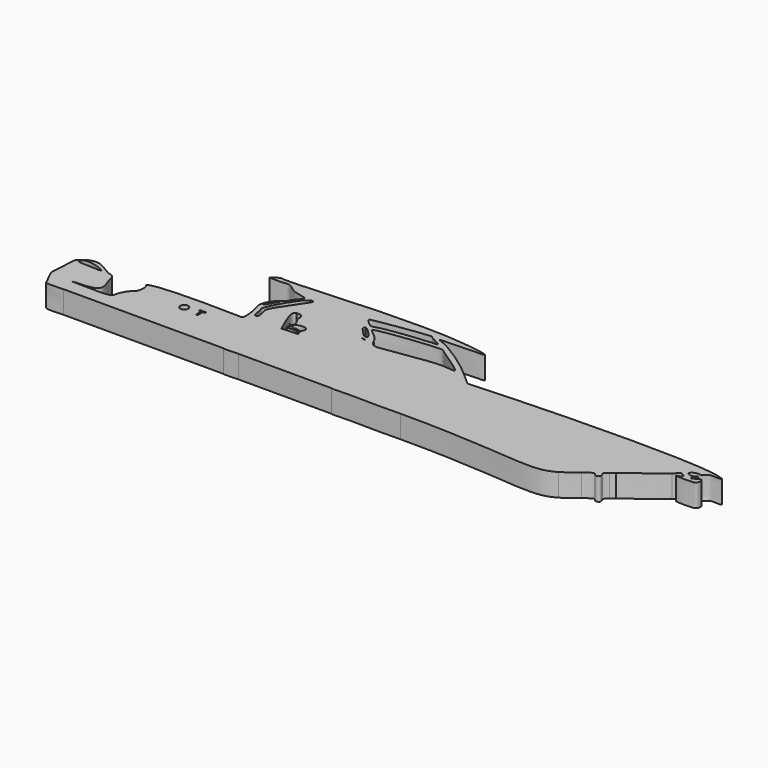
from build123d import *

# Parameters (mm, degrees)
F0_R     = 1.735828002
F1_DEPTH = 9.906


# Not quite as in the source:
# - a feature names something its author has since deleted; it is built from what else it names


with BuildPart() as f1:
    # F0 (on Top) → F1 (new body)
    with BuildSketch(Plane.XY):
        with BuildLine():
            add(Edge.make_bspline(
                [(181.7070857524, 12.9581492726), (181.3160846649, 13.0694763777), (171.7126869599, 17.0451590909), (106.450533251, 15.778155012), (69.6900859475, 13.5057969019)],
                knots=[0.0181687305, 0.0181687305, 0.0181687305, 0.0181687305, 0.0992372423, 0.5806503873, 0.5806503873, 0.5806503873, 0.5806503873], degree=3))
            add(Edge.make_bspline(
                [(69.6900859475, 13.5057969019), (46.0973907721, 12.0474073514), (24.7516413203, 9.403863054), (23.4549589902, 8.8764271796), (19.9190564454, 8.5168434307)],
                knots=[0.5806503873, 0.5806503873, 0.5806503873, 0.5806503873, 0.8896192497, 1, 1, 1, 1], degree=3))
            add(Edge.make_bspline(
                [(19.9190564454, 8.5168434307), (17.4676650102, 8.1993707105), (12.0162404463, 7.4933722476), (-0.135088308, 4.7670167299), (-6.1064609958, 3.2006267697), (-14.1477540249, 3.5424096416), (-21.6224677861, 3.7269103341)],
                knots=[0, 0, 0, 0, 0.0359936003, 0.0800441177, 0.1106409376, 0.1609466089, 0.1609466089, 0.1609466089, 0.1609466089], degree=3))
            add(Edge.make_bspline(
                [(-21.6224677861, 3.7269103341), (-32.9219585505, 4.005819191), (-55.8180186536, 4.2959920551), (-62.3599502161, 2.2052144497), (-62.1269792318, 1.8509117654)],
                knots=[0.1609466089, 0.1609466089, 0.1609466089, 0.1609466089, 0.236993463, 0.2636435799, 0.2636435799, 0.2636435799, 0.2636435799], degree=3))
            add(Edge.make_bspline(
                [(-62.1269792318, 1.8509117654), (-62.1143161054, 1.8367462376), (-62.101652979, 1.8225807098), (-62.0890020197, 1.8083766563)],
                knots=[0, 0, 0, 0, 0.0040737181, 0.0040737181, 0.0040737181, 0.0040737181], degree=3))
            add(Edge.make_bspline(
                [(-62.0890020197, 1.8083766563), (-61.861903726, 1.6076355151), (-60.1495223277, 1.3262390965), (-58.7832820227, 0.8461268043), (-52.5991049945, 0.8259101603), (-44.5873551936, 0.8045360783), (-38.4716986515, 0.9143963036), (-28.4774091761, 1.0996765249), (-16.1932718144, 0.7142595445), (-10.6895341404, 0.9946984772), (-5.449048277, 0.7670292415), (-2.858249547, 1.3382218789), (0.1983725594, 2.3648289955), (1.4864198165, 2.7889108751)],
                knots=[0.2647332889, 0.2647332889, 0.2647332889, 0.2647332889, 0.2804985871, 0.296751932, 0.3273978904, 0.3637260288, 0.3948079699, 0.4350461602, 0.4794644674, 0.5096583468, 0.5375063976, 0.558553087, 0.585278667, 0.585278667, 0.585278667, 0.585278667], degree=3))
            add(Edge.make_bspline(
                [(1.4864198165, 2.7889108751), (2.5730539489, 3.1466786843), (4.4584634209, 3.748123171), (10.8733523881, 4.5985160145), (15.272056911, 5.6548268597), (21.1046291923, 6.5191676625), (28.0641113783, 7.5548859125), (52.7585985721, 10.7246110457), (65.7444362113, 10.6342542254), (72.0763572093, 11.8721236252), (132.1513691778, 12.467602904), (181.7070857524, 12.9581492726)],
                knots=[0.585278667, 0.585278667, 0.585278667, 0.585278667, 0.6078251436, 0.6393387701, 0.6669634416, 0.6961942967, 0.7301717216, 0.793934581, 0.8383697732, 0.8667529058, 0.9998969364, 0.9998969364, 0.9998969364, 0.9998969364], degree=3))
        make_face()
        with BuildLine():
            add(Edge.make_bspline(
                [(69.6900859475, 13.5057969019), (46.0973907721, 12.0474073514), (24.7516413203, 9.403863054), (23.4549589902, 8.8764271796), (19.9190564454, 8.5168434307)],
                knots=[0.5806503873, 0.5806503873, 0.5806503873, 0.5806503873, 0.8896192497, 1, 1, 1, 1], degree=3))
            add(Edge.make_bspline(
                [(-32.5296521187, 32.6141417027), (-31.3157910097, 33.5724732534), (-29.3571477605, 35.1188029908), (-27.6202321809, 34.0767531544), (0.8249259172, 36.2700535088), (31.2175375693, 37.1804566476), (49.4536321074, 36.4065733844), (69.3127565879, 32.985000615), (38.7618020948, 33.6435412252), (44.2668843403, 32.1137581005), (51.7651660713, 27.9376072981), (61.6112530423, 20.8457781991), (67.040172836, 15.8285102723), (69.6900859475, 13.5057969019)],
                knots=[0, 0, 0, 0, 0.0527292582, 0.0850128218, 0.2240344771, 0.3801343496, 0.5042178826, 0.5822497204, 0.6998266016, 0.7329381334, 0.8150611757, 0.9107169826, 1, 1, 1, 1], degree=3))
            add(Edge.make_bspline(
                [(-32.5296521187, 32.6141417027), (-30.3104056847, 32.52847609), (-26.5690998673, 32.391920198), (-23.2049727281, 33.2819990285), (-19.7617512793, 28.9993191577), (-10.3988767952, 28.7616312209), (-16.2720736116, 25.3132861108), (-16.9129986316, 22.6762704551)],
                knots=[0, 0, 0, 0, 0.2160762386, 0.3662971417, 0.569378152, 0.7796526031, 1, 1, 1, 1], degree=3))
            add(Edge.make_bspline(
                [(-16.9129986316, 22.6762704551), (-17.8467477386, 22.1680560361), (-19.9763271995, 21.0089834539), (-23.3696805255, 15.5020605961), (-21.7713441225, 12.3045577284), (-20.779820899, 4.7533250441), (-21.4380773918, 3.9515133273), (-21.6224677861, 3.7269103341)],
                knots=[0, 0, 0, 0, 0.1877547788, 0.4282078748, 0.6241699663, 0.8947227276, 1, 1, 1, 1], degree=3))
            add(Edge.make_bspline(
                [(19.9190564454, 8.5168434307), (17.4676650102, 8.1993707105), (12.0162404463, 7.4933722476), (-0.135088308, 4.7670167299), (-6.1064609958, 3.2006267697), (-14.1477540249, 3.5424096416), (-21.6224677861, 3.7269103341)],
                knots=[0, 0, 0, 0, 0.0359936003, 0.0800441177, 0.1106409376, 0.1609466089, 0.1609466089, 0.1609466089, 0.1609466089], degree=3))
        make_face()
        with BuildLine():
            add(Edge.make_bspline(
                [(-8.7680807337, 17.8092923015), (-8.3866222979, 17.8483506489), (-7.546092961, 17.9344142503), (-5.9981024532, 17.2405624552), (-5.6060574812, 15.7239200529), (-6.0102153242, 14.5268353778), (-5.4550952735, 13.7705655392), (-4.6619934349, 12.9765246302), (-4.4702294547, 12.3041590957), (-4.0660592451, 10.8605465604), (-4.3298750077, 9.9418295588), (-5.4584476986, 9.754342472), (-5.6748329949, 10.4291802539), (-5.6347727128, 9.3913742433), (-4.3029010056, 9.7861895365), (-4.3140752557, 8.9878988444), (-4.4250907254, 8.1865468653), (-5.1640550787, 7.5215406766), (-4.3832359422, 7.2748261031), (-3.3321553041, 7.4747711988), (-2.8663373676, 7.4992743174), (-2.115136075, 7.4933709617), (-0.8968103525, 7.1797893281), (-1.5445606345, 7.8573288432), (-1.310513294, 9.0220769068), (-2.6227539696, 8.3145975273), (-3.1977834194, 8.2778539141), (-3.4696750478, 8.9956573412), (-4.0448585774, 9.7693814037), (-3.9314235683, 10.394370376), (-3.4871454114, 10.8062850186), (-2.8829533176, 11.0326311001), (-2.4154737172, 11.2246835665), (-2.3047583969, 11.3243672691), (-1.5621432493, 11.3791968524), (-0.7704961294, 11.3668207714), (0.0011303932, 11.2391718235), (0.2761138653, 11.255904495), (0.9514057607, 11.01202914), (1.2073443869, 10.382397098), (1.4002015739, 9.6657434855), (1.0307265988, 8.9530975397), (0.7733677818, 8.2984308224), (-0.4727618848, 7.7586873364), (-0.8225833851, 9.2751421466), (-0.4934208188, 7.4734539438), (0.0075581501, 7.445925416), (0.3338729219, 7.68534912), (0.9549221847, 7.2664605316), (1.3294265015, 6.722294157), (1.2187918234, 6.2131527361), (1.1623987395, 5.9606525059)],
                knots=[0, 0, 0, 0, 0.0260454786, 0.0555593992, 0.0840154219, 0.1096289478, 0.1317188239, 0.1562843989, 0.1764181206, 0.2050873592, 0.2270500346, 0.249871093, 0.2633196669, 0.2802385774, 0.3041836822, 0.3215813241, 0.3439096138, 0.3640338166, 0.3813082826, 0.4062842171, 0.4223932343, 0.4439778086, 0.4659830297, 0.4836895774, 0.5050499879, 0.5297363334, 0.5468542516, 0.5664129357, 0.5896734041, 0.6073348608, 0.6252199, 0.644737738, 0.6610014027, 0.6698170215, 0.6893495641, 0.7117052382, 0.7320089542, 0.7446274286, 0.7635758386, 0.7829107313, 0.8029010202, 0.8234292288, 0.84378532, 0.8679512846, 0.8872861973, 0.9123156375, 0.9274517817, 0.9412478508, 0.9605987473, 0.9795496341, 1, 1, 1, 1], degree=3))
            add(Edge.make_bspline(
                [(1.1623987395, 5.9606525059), (-1.3945692664, 5.7893390901), (-5.1543167158, 5.7216326818), (-5.4948480663, 5.4527658301), (-5.6129922159, 5.3594848141)],
                knots=[0.9337593868, 0.9337593868, 0.9337593868, 0.9337593868, 0.9769868279, 1, 1, 1, 1], degree=3))
            add(Edge.make_bspline(
                [(-8.7680807337, 17.8092923015), (-9.1752028405, 17.6145650541), (-10.8178823014, 16.8288684671), (-7.8473254678, 10.2830134292), (-5.6129922159, 5.3594848141)],
                knots=[0, 0, 0, 0, 0.2478402613, 1, 1, 1, 1], degree=3))
        make_face(mode=Mode.SUBTRACT)
        with BuildLine():
            add(Edge.make_bspline(
                [(-18.4361021966, 21.1632531136), (-18.5670530022, 21.2586161996), (-21.070472051, 18.5655291506), (-22.3743986232, 16.3744597495), (-21.4413586586, 15.2038485553), (-20.4225931001, 17.854661305), (-18.2993558507, 21.0636695068), (-18.4361021966, 21.1632531136)],
                knots=[0, 0, 0, 0, 0.2351165364, 0.4465883524, 0.5497009663, 0.7544778204, 1, 1, 1, 1], degree=3))
        make_face(mode=Mode.SUBTRACT)
        with BuildLine():
            add(Edge.make_bspline(
                [(-9.7060799599, 27.9816947877), (-9.8874931048, 28.2447168603), (-12.368524278, 29.356752937), (-21.4951287489, 13.0755897254), (-19.6376283471, 12.2112957368), (-19.6141174394, 7.2221985209), (-17.0553430775, 7.6758488961), (-18.6586504228, 11.9438536073), (-18.5103546144, 13.6291611502), (-17.1677183959, 16.6289965217), (-10.000495834, 26.8513547323), (-9.5698072007, 27.7841195592), (-9.7060799599, 27.9816947877)],
                knots=[0, 0, 0, 0, 0.0653917324, 0.2773427404, 0.3459565689, 0.4503618884, 0.5044288692, 0.6067460895, 0.6730479064, 0.7686451707, 0.9508794591, 1, 1, 1, 1], degree=3))
        make_face(mode=Mode.SUBTRACT)
        with BuildLine():
            add(Edge.make_bspline(
                [(22.0193362931, 17.0219166161), (21.0430994165, 17.2670474431), (19.9439292923, 17.5707458095), (19.3718951195, 17.5534747541)],
                knots=[0.6042790893, 0.6042790893, 0.6042790893, 0.6042790893, 0.632909986, 0.632909986, 0.632909986, 0.632909986], degree=3))
            add(Edge.make_bspline(
                [(22.0193362931, 17.0219166161), (21.930461642, 16.7429022187), (20.6518410174, 17.150070539), (19.3718951195, 17.5534747541)],
                knots=[0.9338982102, 0.9338982102, 0.9338982102, 0.9338982102, 1, 1, 1, 1], degree=3))
        make_face(mode=Mode.SUBTRACT)
        with BuildLine():
            add(Edge.make_bspline(
                [(19.099231914, 19.6574293824), (19.2141128722, 19.559261403), (19.3324185741, 19.4665098594), (19.4542166063, 19.3811532624)],
                knots=[0.4773801215, 0.4773801215, 0.4773801215, 0.4773801215, 0.5030785781, 0.5030785781, 0.5030785781, 0.5030785781], degree=3))
            add(Edge.make_bspline(
                [(16.2104386836, 24.2807362229), (15.7704996157, 24.2210769069), (16.1269574289, 22.4635564191), (17.0786160293, 22.2094376386), (18.2129434355, 20.4147798645), (19.099231914, 19.6574293824)],
                knots=[0, 0, 0, 0, 0.1478459221, 0.2791205811, 0.4773801215, 0.4773801215, 0.4773801215, 0.4773801215], degree=3))
            add(Edge.make_bspline(
                [(21.0577676507, 18.8489194134), (21.20328979, 18.8904985397), (21.8588734633, 19.6430869693), (17.1846356138, 24.4128452505), (16.2104386836, 24.2807362229)],
                knots=[0.6228285443, 0.6228285443, 0.6228285443, 0.6228285443, 0.672611382, 1, 1, 1, 1], degree=3))
            add(Edge.make_bspline(
                [(19.649869615, 19.2525507144), (20.1684843746, 18.9343377038), (20.7473442621, 18.7602240898), (21.0577676507, 18.8489194134)],
                knots=[0.5166333136, 0.5166333136, 0.5166333136, 0.5166333136, 0.6228285443, 0.6228285443, 0.6228285443, 0.6228285443], degree=3))
            add(Edge.make_bspline(
                [(19.4542166063, 19.3811532624), (19.5194574132, 19.3351449211), (19.5846240735, 19.2921451484), (19.649869615, 19.2525507144)],
                knots=[0.4893319279, 0.4893319279, 0.4893319279, 0.4893319279, 0.4932270857, 0.4932270857, 0.4932270857, 0.4932270857], degree=3))
        make_face(mode=Mode.SUBTRACT)
        with BuildLine():
            add(Edge.make_bspline(
                [(26.768874377, 15.5890742317), (28.477421113, 14.8122982972), (35.2147378262, 16.493420054), (41.3114742367, 16.8146107371), (54.2220403717, 19.4096476067), (64.7203055195, 16.7217366675), (47.1864971217, 27.407686439), (47.969181218, 28.4052858834), (17.3145197031, 25.37667601), (19.9733974533, 23.3131590908), (22.3191658115, 21.5089275881), (24.8989437371, 18.7282663545), (25.6097683501, 16.1160517198), (26.768874377, 15.5890742317)],
                knots=[0, 0, 0, 0, 0.0984646732, 0.1912591061, 0.323936191, 0.3995561971, 0.5344920224, 0.5848516391, 0.76862153, 0.8014841712, 0.8639750777, 0.9331999566, 1, 1, 1, 1], degree=3))
        make_face(mode=Mode.SUBTRACT)
        with BuildLine():
            add(Edge.make_bspline(
                [(13.7598691508, 29.2401816696), (14.0794886419, 28.511657453), (16.931970818, 25.6172264089), (19.0667686569, 26.8110867482), (27.6858636418, 28.3987828014), (40.9320979411, 29.6761274961), (44.8001711563, 29.781861299), (38.0692510724, 32.9302009921), (38.7545990359, 33.7239035632), (14.6777023437, 30.2669926278), (13.5969193313, 29.6116011009), (13.7598691508, 29.2401816696)],
                knots=[0, 0, 0, 0, 0.1009240569, 0.1708567082, 0.3169576193, 0.502818054, 0.5609304523, 0.6778465933, 0.710253389, 0.9485464519, 1, 1, 1, 1], degree=3))
        make_face(mode=Mode.SUBTRACT)
        with BuildLine():
            add(Edge.make_bspline(
                [(181.7070857524, 12.9581492726), (181.7454456589, 12.958528993), (181.7838055875, 12.9589087131), (181.8221655209, 12.9592884332)],
                knots=[0.9998969364, 0.9998969364, 0.9998969364, 0.9998969364, 1, 1, 1, 1], degree=3))
            add(Edge.make_bspline(
                [(181.8221655209, 12.9592884332), (181.8324633094, 12.9314378649), (181.7947152553, 12.9331991147), (181.7070857524, 12.9581492726)],
                knots=[0, 0, 0, 0, 0.0181687305, 0.0181687305, 0.0181687305, 0.0181687305], degree=3))
        make_face()
        with BuildLine():
            add(Edge.make_bspline(
                [(181.8221655209, 12.9592884332), (181.8324633094, 12.9314378649), (181.7947152553, 12.9331991147), (181.7070857524, 12.9581492726)],
                knots=[0, 0, 0, 0, 0.0181687305, 0.0181687305, 0.0181687305, 0.0181687305], degree=3))
            add(Edge.make_bspline(
                [(1.4864198165, 2.7889108751), (2.5730539489, 3.1466786843), (4.4584634209, 3.748123171), (10.8733523881, 4.5985160145), (15.272056911, 5.6548268597), (21.1046291923, 6.5191676625), (28.0641113783, 7.5548859125), (52.7585985721, 10.7246110457), (65.7444362113, 10.6342542254), (72.0763572093, 11.8721236252), (132.1513691778, 12.467602904), (181.7070857524, 12.9581492726)],
                knots=[0.585278667, 0.585278667, 0.585278667, 0.585278667, 0.6078251436, 0.6393387701, 0.6669634416, 0.6961942967, 0.7301717216, 0.793934581, 0.8383697732, 0.8667529058, 0.9998969364, 0.9998969364, 0.9998969364, 0.9998969364], degree=3))
            add(Edge.make_bspline(
                [(1.4864198165, 2.7889108751), (4.2205646602, 2.8036473169), (10.895287819, 2.8396058817), (29.9301094809, 2.4768207335), (49.5703435401, 4.0355304108), (76.9900908256, 3.2337996187), (130.8518333078, 4.4349005585), (166.0121836622, 5.2259781687)],
                knots=[0, 0, 0, 0, 0.1142026761, 0.2787903661, 0.4447220453, 0.6374813456, 1, 1, 1, 1], degree=3))
            add(Edge.make_bspline(
                [(181.8221655209, 12.9592884332), (181.8784118357, 12.8071691869), (182.1168141897, 12.1624054099), (177.2940506946, 12.8181824665), (176.323693659, 11.7841511594), (174.4359593488, 10.2223841308), (172.9776336012, 11.1250817767), (169.0091153843, 9.0901845191), (172.9265663934, 7.3718884696), (173.9202331987, 9.1733929637), (175.2498946984, 8.6368197357), (173.5447616732, 7.6949049995), (173.1379225552, 7.5029866377), (173.2602047255, 6.7080592442), (173.4359940525, 6.0179457322), (177.6085839303, 9.5031250099), (177.3260097226, 4.9015096015), (175.0945252898, 4.4842240475), (167.2377249395, 4.5555836395), (168.8205212842, 5.2477294336), (170.1461048916, 5.0856746733), (170.3461464599, 7.0417235878), (168.7632613231, 6.8991093543), (168.2757313043, 7.9553484486), (167.652880774, 6.7273321612), (166.0121836622, 5.2259781687)],
                knots=[0, 0, 0, 0, 0.0123247893, 0.0522391341, 0.0772012243, 0.1051179002, 0.1304384627, 0.1635602749, 0.1943191106, 0.2203426345, 0.2359897164, 0.2598670338, 0.273320428, 0.2900500035, 0.3014773465, 0.3389355156, 0.369061601, 0.4002658601, 0.4502194286, 0.4648952703, 0.4868630471, 0.5087361933, 0.530592032, 0.5456456248, 0.5810716893, 0.5810716893, 0.5810716893, 0.5810716893], degree=3))
        make_face()
        with BuildLine():
            add(Edge.make_bspline(
                [(1.4864198165, 2.7889108751), (4.2205646602, 2.8036473169), (10.895287819, 2.8396058817), (29.9301094809, 2.4768207335), (49.5703435401, 4.0355304108), (76.9900908256, 3.2337996187), (130.8518333078, 4.4349005585), (166.0121836622, 5.2259781687)],
                knots=[0, 0, 0, 0, 0.1142026761, 0.2787903661, 0.4447220453, 0.6374813456, 1, 1, 1, 1], degree=3))
            add(Edge.make_bspline(
                [(-62.0890020197, 1.8083766563), (-61.861903726, 1.6076355151), (-60.1495223277, 1.3262390965), (-58.7832820227, 0.8461268043), (-52.5991049945, 0.8259101603), (-44.5873551936, 0.8045360783), (-38.4716986515, 0.9143963036), (-28.4774091761, 1.0996765249), (-16.1932718144, 0.7142595445), (-10.6895341404, 0.9946984772), (-5.449048277, 0.7670292415), (-2.858249547, 1.3382218789), (0.1983725594, 2.3648289955), (1.4864198165, 2.7889108751)],
                knots=[0.2647332889, 0.2647332889, 0.2647332889, 0.2647332889, 0.2804985871, 0.296751932, 0.3273978904, 0.3637260288, 0.3948079699, 0.4350461602, 0.4794644674, 0.5096583468, 0.5375063976, 0.558553087, 0.585278667, 0.585278667, 0.585278667, 0.585278667], degree=3))
            add(Edge.make_bspline(
                [(-62.0890020197, 1.8083766563), (-61.8617706553, 1.5532492479), (-61.2363578093, 0.8039040443), (-61.1708004572, -3.2918532801), (-63.6717034466, -4.7618703301), (-66.3410506075, -9.4747360166), (-65.5308334758, -13.0903445127), (-83.1668567567, -11.6324037514), (-83.6185440421, -12.0004769415)],
                knots=[0.0040737181, 0.0040737181, 0.0040737181, 0.0040737181, 0.0772441787, 0.209002126, 0.3271483234, 0.4831134652, 0.5924502027, 0.872940585, 0.872940585, 0.872940585, 0.872940585], degree=3))
            add(Edge.make_bspline(
                [(-83.6185440421, -12.0004769415), (-83.6878383721, -12.056943851), (-83.041986797, -12.3221575597), (-83.5031714482, -13.1574132129), (-83.8081687689, -13.7097965926)],
                knots=[0.872940585, 0.872940585, 0.872940585, 0.872940585, 0.9159712253, 1, 1, 1, 1], degree=3))
            add(Edge.make_bspline(
                [(150.8671206532, -6.3339171309), (149.9451168632, -6.3093856293), (129.0676805339, -7.7990941469), (75.8255428962, -11.4168639952), (40.6726759359, -14.0739481615), (-5.1835527569, -14.0668096823), (-32.3090070132, -13.611541778), (-54.4750501881, -13.8010523094), (-80.0915545979, -12.8371898834), (-83.8081687689, -13.7097965926)],
                knots=[0.0068929718, 0.0068929718, 0.0068929718, 0.0068929718, 0.0424850168, 0.1304200504, 0.2004080673, 0.2762381099, 0.3349013753, 0.3910747276, 0.4502039223, 0.4502039223, 0.4502039223, 0.4502039223], degree=3))
            add(Edge.make_bspline(
                [(166.0121836622, 5.2259781687), (162.8653802069, 2.3464302636), (155.2910613494, -2.8857498256), (150.8671206532, -6.3339171309)],
                knots=[0.5810716893, 0.5810716893, 0.5810716893, 0.5810716893, 0.6490177235, 0.6490177235, 0.6490177235, 0.6490177235], degree=3))
        make_face()
        with Locations((-41.5836200118, -2.8440221213)):
            Circle(F0_R, mode=Mode.SUBTRACT)
        Polygon((-35.9781831503, -1.7277105944), (-35.9781831503, -1.1352393303), (-33.4241501987, -1.1401575757), (-33.4177240729, -1.7587322509), (-34.3434922397, -1.7651341623), (-34.3650206923, -4.5761046931), (-35.0652709603, -4.5950240456), (-35.0776910782, -1.7277105944), align=None, mode=Mode.SUBTRACT)
        with BuildLine():
            add(Edge.make_bspline(
                [(-62.1269792318, 1.8509117654), (-62.1143161054, 1.8367462376), (-62.101652979, 1.8225807098), (-62.0890020197, 1.8083766563)],
                knots=[0, 0, 0, 0, 0.0040737181, 0.0040737181, 0.0040737181, 0.0040737181], degree=3))
            add(Edge.make_bspline(
                [(-62.1269792318, 1.8509117654), (-62.1174531732, 1.8364245186), (-62.1046992206, 1.8222520315), (-62.0890020197, 1.8083766563)],
                knots=[0.2636435799, 0.2636435799, 0.2636435799, 0.2636435799, 0.2647332889, 0.2647332889, 0.2647332889, 0.2647332889], degree=3))
        make_face()
        with BuildLine():
            add(Edge.make_bspline(
                [(150.8671206532, -6.3339171309), (150.8358641495, -6.358279495), (150.8047649082, -6.3825528038), (150.773825602, -6.4067355982)],
                knots=[0.6490177235, 0.6490177235, 0.6490177235, 0.6490177235, 0.6494977832, 0.6494977832, 0.6494977832, 0.6494977832], degree=3))
            add(Edge.make_bspline(
                [(150.8671206532, -6.3339171309), (149.9451168632, -6.3093856293), (129.0676805339, -7.7990941469), (75.8255428962, -11.4168639952), (40.6726759359, -14.0739481615), (-5.1835527569, -14.0668096823), (-32.3090070132, -13.611541778), (-54.4750501881, -13.8010523094), (-80.0915545979, -12.8371898834), (-83.8081687689, -13.7097965926)],
                knots=[0.0068929718, 0.0068929718, 0.0068929718, 0.0068929718, 0.0424850168, 0.1304200504, 0.2004080673, 0.2762381099, 0.3349013753, 0.3910747276, 0.4502039223, 0.4502039223, 0.4502039223, 0.4502039223], degree=3))
            add(Edge.make_bspline(
                [(-83.8081687689, -13.7097965926), (-84.6369010791, -13.9043708316), (-84.9972691043, -14.1669073509), (-84.9167108536, -14.4772501662)],
                knots=[0.4502039223, 0.4502039223, 0.4502039223, 0.4502039223, 0.4633885769, 0.4633885769, 0.4633885769, 0.4633885769], degree=3))
            add(Edge.make_bspline(
                [(-84.9167108536, -14.4772501662), (-84.7138619392, -14.6725496732), (-84.5185424306, -14.8710134926), (-84.3328175272, -15.0689651244)],
                knots=[0, 0, 0, 0, 0.1476817979, 0.1476817979, 0.1476817979, 0.1476817979], degree=3))
            add(Edge.make_bspline(
                [(-84.3328175272, -15.0689651244), (-83.9927052357, -15.2743058553), (-82.0006271924, -16.0869905544), (-75.7367051465, -15.2762348592), (-58.1178632592, -15.5293752531), (-38.2276766459, -16.077011161), (-33.0082327019, -15.9831740161), (-4.9036389077, -16.0144239851), (11.3771966117, -16.0352215062), (71.5506366852, -14.0905273715), (94.855980366, -11.5853831358), (103.7875194567, -11.2072546361), (148.042941917, -6.8791730342), (150.773825602, -6.4067355982)],
                knots=[0.4714918964, 0.4714918964, 0.4714918964, 0.4714918964, 0.4801500531, 0.5092457996, 0.558426584, 0.6081692403, 0.6357120753, 0.6928549825, 0.7434689124, 0.8312284931, 0.8846782089, 0.9241105362, 0.9997444898, 0.9997444898, 0.9997444898, 0.9997444898], degree=3))
        make_face()
        with BuildLine():
            add(Edge.make_bspline(
                [(150.8005982928, -6.4020289535), (151.0332048701, -6.360438073), (151.0456815115, -6.3386680506), (150.8671206532, -6.3339171309)],
                knots=[0, 0, 0, 0, 0.0068929718, 0.0068929718, 0.0068929718, 0.0068929718], degree=3))
            add(Edge.make_bspline(
                [(150.8671206532, -6.3339171309), (150.8358641495, -6.358279495), (150.8047649082, -6.3825528038), (150.773825602, -6.4067355982)],
                knots=[0.6490177235, 0.6490177235, 0.6490177235, 0.6490177235, 0.6494977832, 0.6494977832, 0.6494977832, 0.6494977832], degree=3))
            add(Edge.make_bspline(
                [(150.773825602, -6.4067355982), (150.7830512011, -6.4051395879), (150.791975982, -6.4035706533), (150.8005982928, -6.4020289535)],
                knots=[0.9997444898, 0.9997444898, 0.9997444898, 0.9997444898, 1, 1, 1, 1], degree=3))
        make_face()
        with BuildLine():
            add(Edge.make_bspline(
                [(-83.6185440421, -12.0004769415), (-83.6878383721, -12.056943851), (-83.041986797, -12.3221575597), (-83.5031714482, -13.1574132129), (-83.8081687689, -13.7097965926)],
                knots=[0.872940585, 0.872940585, 0.872940585, 0.872940585, 0.9159712253, 1, 1, 1, 1], degree=3))
            add(Edge.make_bspline(
                [(-83.6185440421, -12.0004769415), (-83.0740160087, -11.5131255971), (-69.1822427079, -12.6336350445), (-75.6026010724, -2.1341319734), (-74.3979178815, -0.0363802838), (-77.8765454888, 0.7573231123)],
                knots=[0, 0, 0, 0, 0.3934519621, 0.7281196259, 1, 1, 1, 1], degree=3))
            add(Edge.make_bspline(
                [(-77.8765454888, 0.7573231123), (-78.6146260032, 1.1131316014), (-79.7527983343, 1.8416604009), (-83.3603098815, 4.0141024595), (-86.0361955364, 4.8071239155), (-89.0577730813, 4.19382815), (-91.622500244, 2.3560975429), (-93.0282857603, 0.8473538246), (-92.9040429007, -2.9442481756), (-93.0456637378, -6.8325637035), (-93.8186976488, -10.6780024025), (-92.261573742, -13.6256031139), (-90.2656212016, -17.2398359526), (-90.3162580306, -18.7953536323), (-82.5034658756, -18.2195524685), (-82.368550436, -18.2317357257), (-82.3523029633, -18.2346555499)],
                knots=[0, 0, 0, 0, 0.0627443894, 0.1474187464, 0.2176997034, 0.2898115377, 0.363582417, 0.4214715407, 0.5006663333, 0.5856458823, 0.666188716, 0.7436240317, 0.8271254841, 0.8726215951, 0.9854356816, 1, 1, 1, 1], degree=3))
            add(Edge.make_bspline(
                [(-84.3328175272, -15.0689651244), (-83.8111744216, -15.6249492819), (-82.8948242675, -16.7590880701), (-82.4912554681, -17.5322230476), (-82.3523029633, -18.2346555499)],
                knots=[0.1476817979, 0.1476817979, 0.1476817979, 0.1476817979, 0.5624737309, 1, 1, 1, 1], degree=3))
            add(Edge.make_bspline(
                [(-84.9167108536, -14.4772501662), (-84.8671995649, -14.6679875842), (-84.6511345369, -14.8767831624), (-84.3328175272, -15.0689651244)],
                knots=[0.4633885769, 0.4633885769, 0.4633885769, 0.4633885769, 0.4714918964, 0.4714918964, 0.4714918964, 0.4714918964], degree=3))
            add(Edge.make_bspline(
                [(-83.8081687689, -13.7097965926), (-84.6369010791, -13.9043708316), (-84.9972691043, -14.1669073509), (-84.9167108536, -14.4772501662)],
                knots=[0.4502039223, 0.4502039223, 0.4502039223, 0.4502039223, 0.4633885769, 0.4633885769, 0.4633885769, 0.4633885769], degree=3))
        make_face()
        with BuildLine():
            add(Edge.make_bspline(
                [(-80.9516832232, 0.7573231123), (-80.876809325, 0.1354285261), (-88.3160753781, 0.9633882243), (-91.8051389553, 0.6728053118), (-89.6347601206, 4.557778789), (-81.0335859871, 1.4375987042), (-80.9516832232, 0.7573231123)],
                knots=[0, 0, 0, 0, 0.300587952, 0.4939423969, 0.6711940392, 1, 1, 1, 1], degree=3))
        make_face(mode=Mode.SUBTRACT)
        with BuildLine():
            add(Edge.make_bspline(
                [(150.773825602, -6.4067355982), (150.1262005755, -6.9129325614), (149.5486516192, -7.379470369), (149.0656908578, -7.7929682632)],
                knots=[0.6494977832, 0.6494977832, 0.6494977832, 0.6494977832, 0.6595464458, 0.6595464458, 0.6595464458, 0.6595464458], degree=3))
            add(Edge.make_bspline(
                [(-84.3328175272, -15.0689651244), (-83.9927052357, -15.2743058553), (-82.0006271924, -16.0869905544), (-75.7367051465, -15.2762348592), (-58.1178632592, -15.5293752531), (-38.2276766459, -16.077011161), (-33.0082327019, -15.9831740161), (-4.9036389077, -16.0144239851), (11.3771966117, -16.0352215062), (71.5506366852, -14.0905273715), (94.855980366, -11.5853831358), (103.7875194567, -11.2072546361), (148.042941917, -6.8791730342), (150.773825602, -6.4067355982)],
                knots=[0.4714918964, 0.4714918964, 0.4714918964, 0.4714918964, 0.4801500531, 0.5092457996, 0.558426584, 0.6081692403, 0.6357120753, 0.6928549825, 0.7434689124, 0.8312284931, 0.8846782089, 0.9241105362, 0.9997444898, 0.9997444898, 0.9997444898, 0.9997444898], degree=3))
            add(Edge.make_bspline(
                [(-84.3328175272, -15.0689651244), (-83.8111744216, -15.6249492819), (-82.8948242675, -16.7590880701), (-82.4912554681, -17.5322230476), (-82.3523029633, -18.2346555499)],
                knots=[0.1476817979, 0.1476817979, 0.1476817979, 0.1476817979, 0.5624737309, 1, 1, 1, 1], degree=3))
            add(Edge.make_bspline(
                [(-12.012616726, -18.2346555499), (-35.4591788051, -18.2346555499), (-58.9057408842, -18.2346555499), (-82.3523029633, -18.2346555499)],
                knots=[0, 0, 0, 0, 70.3396862373, 70.3396862373, 70.3396862373, 70.3396862373], degree=3))
            add(Edge.make_bspline(
                [(-12.012616726, -18.2346555499), (-11.9112376122, -18.0097504648), (-9.2297296101, -17.249512571), (-8.5133003062, -17.1385317605), (-6.6794104422, -17.1280550014), (-5.5318949744, -17.1214994043)],
                knots=[0.723140227, 0.723140227, 0.723140227, 0.723140227, 0.8275161404, 0.8920720919, 1, 1, 1, 1], degree=3))
            add(Edge.make_bspline(
                [(-5.5318949744, -17.1214994043), (-5.5176828367, -17.4925514528), (-5.5034706938, -17.8636035014), (-5.4892585561, -18.2346555499)],
                knots=[0, 0, 0, 0, 1.1139723823, 1.1139723823, 1.1139723823, 1.1139723823], degree=3))
            add(Edge.make_bspline(
                [(35.3563390724, -18.2346555499), (24.7668170063, -18.272613468), (7.1827417938, -18.3356432142), (-1.2190889389, -18.0846871761), (-5.4892585561, -18.2346555499)],
                knots=[0, 0, 0, 0, 0.33800155, 0.5612571221, 0.5612571221, 0.5612571221, 0.5612571221], degree=3))
            add(Edge.make_bspline(
                [(65.6281337194, -18.2346555499), (58.5311162328, -18.6015132536), (45.3210777903, -17.8463649568), (35.2723890544, -18.5648869649), (35.3563390724, -18.2346555499)],
                knots=[0.5617491704, 0.5617491704, 0.5617491704, 0.5617491704, 0.7184550903, 0.8107984489, 0.8107984489, 0.8107984489, 0.8107984489], degree=3))
            add(Edge.make_bspline(
                [(149.0656908575, -7.7929682623), (148.680018805, -7.7692609038), (146.0188251162, -7.7112684335), (111.4024955856, -12.3068345195), (84.3744740498, -15.5884842443), (72.0197005784, -17.9042638684), (65.6281337194, -18.2346555499)],
                knots=[0.006710192, 0.006710192, 0.006710192, 0.006710192, 0.0465203096, 0.2392235246, 0.4206199755, 0.5617491704, 0.5617491704, 0.5617491704, 0.5617491704], degree=3))
        make_face()
        with BuildLine():
            add(Edge.make_bspline(
                [(149.0656908578, -7.7929682632), (148.2775137705, -8.4677840906), (147.1532625722, -9.5863648581), (147.9495626486, -10.0135549698), (148.4031839357, -12.3334511177), (145.999649434, -12.475121483), (145.3914699044, -10.5492060658), (143.0663219155, -12.2768200458), (141.3872051441, -13.606970793)],
                knots=[0.6595464458, 0.6595464458, 0.6595464458, 0.6595464458, 0.6759455537, 0.6939267484, 0.7202153547, 0.7452640055, 0.7685217004, 0.8010181559, 0.8010181559, 0.8010181559, 0.8010181559], degree=3))
            add(Edge.make_bspline(
                [(149.0656908575, -7.7929682623), (148.680018805, -7.7692609038), (146.0188251162, -7.7112684335), (111.4024955856, -12.3068345195), (84.3744740498, -15.5884842443), (72.0197005784, -17.9042638684), (65.6281337194, -18.2346555499)],
                knots=[0.006710192, 0.006710192, 0.006710192, 0.006710192, 0.0465203096, 0.2392235246, 0.4206199755, 0.5617491704, 0.5617491704, 0.5617491704, 0.5617491704], degree=3))
            add(Edge.make_bspline(
                [(112.4813359754, -18.2765493302), (96.9051363175, -18.2379792034), (81.4762857503, -18.1121175646), (65.6281337194, -18.2346555499)],
                knots=[22.5201778066, 22.5201778066, 22.5201778066, 22.5201778066, 69.4440972526, 69.4440972526, 69.4440972526, 69.4440972526], degree=3))
            Line((112.4813359754, -18.2765493302), (141.3872051441, -13.606970793))
        make_face()
        with BuildLine():
            add(Edge.make_bspline(
                [(112.4813359754, -18.2765493302), (96.9051363175, -18.2379792034), (81.4762857503, -18.1121175646), (65.6281337194, -18.2346555499)],
                knots=[22.5201778066, 22.5201778066, 22.5201778066, 22.5201778066, 69.4440972526, 69.4440972526, 69.4440972526, 69.4440972526], degree=3))
            add(Edge.make_bspline(
                [(135.072230972, -18.2346555499), (125.0352715652, -24.1134627301), (115.8400401473, -18.2346555499), (65.6281337194, -18.2346555499)],
                knots=[0.8369193023, 0.8369193023, 0.8369193023, 0.8369193023, 1, 1, 1, 1], degree=3))
            add(Edge.make_bspline(
                [(135.072230972, -18.2346555499), (130.6841629706, -18.2685841121), (126.3282401461, -18.2834694547), (121.9924343306, -18.2864372204)],
                knots=[0, 0, 0, 0, 12.9923885773, 12.9923885773, 12.9923885773, 12.9923885773], degree=3))
            add(Edge.make_bspline(
                [(121.9924343306, -18.2864372204), (118.8128308495, -18.2886135905), (115.6440459341, -18.2843809019), (112.4813359754, -18.2765493302)],
                knots=[12.9923885773, 12.9923885773, 12.9923885773, 12.9923885773, 22.5201778066, 22.5201778066, 22.5201778066, 22.5201778066], degree=3))
        make_face()
        with BuildLine():
            Line((121.9924343306, -18.2864372204), (141.3872051441, -13.606970793))
            Line((141.3872051441, -13.606970793), (112.4813359754, -18.2765493302))
            add(Edge.make_bspline(
                [(121.9924343306, -18.2864372204), (118.8128308495, -18.2886135905), (115.6440459341, -18.2843809019), (112.4813359754, -18.2765493302)],
                knots=[12.9923885773, 12.9923885773, 12.9923885773, 12.9923885773, 22.5201778066, 22.5201778066, 22.5201778066, 22.5201778066], degree=3))
        make_face()
        with BuildLine():
            add(Edge.make_bspline(
                [(141.3872051441, -13.606970793), (139.5321653773, -15.076482964), (137.2818017856, -16.9404746891), (135.072230972, -18.2346555499)],
                knots=[0.8010181559, 0.8010181559, 0.8010181559, 0.8010181559, 0.8369193023, 0.8369193023, 0.8369193023, 0.8369193023], degree=3))
            Line((141.3872051441, -13.606970793), (121.9924343306, -18.2864372204))
            add(Edge.make_bspline(
                [(135.072230972, -18.2346555499), (130.6841629706, -18.2685841121), (126.3282401461, -18.2834694547), (121.9924343306, -18.2864372204)],
                knots=[0, 0, 0, 0, 12.9923885773, 12.9923885773, 12.9923885773, 12.9923885773], degree=3))
        make_face()
        with BuildLine():
            add(Edge.make_bspline(
                [(-12.012616726, -18.2346555499), (-11.9112376122, -18.0097504648), (-9.2297296101, -17.249512571), (-8.5133003062, -17.1385317605), (-6.6794104422, -17.1280550014), (-5.5318949744, -17.1214994043)],
                knots=[0.723140227, 0.723140227, 0.723140227, 0.723140227, 0.8275161404, 0.8920720919, 1, 1, 1, 1], degree=3))
            add(Edge.make_bspline(
                [(-5.4892585561, -18.2346555499), (-8.5855679117, -18.3433979467), (-12.1698519079, -18.5834748543), (-12.012616726, -18.2346555499)],
                knots=[0.5612571221, 0.5612571221, 0.5612571221, 0.5612571221, 0.723140227, 0.723140227, 0.723140227, 0.723140227], degree=3))
            add(Edge.make_bspline(
                [(-5.5318949744, -17.1214994043), (-5.5176828367, -17.4925514528), (-5.5034706938, -17.8636035014), (-5.4892585561, -18.2346555499)],
                knots=[0, 0, 0, 0, 1.1139723823, 1.1139723823, 1.1139723823, 1.1139723823], degree=3))
        make_face()
    extrude(amount=F1_DEPTH)


solid = f1.part
